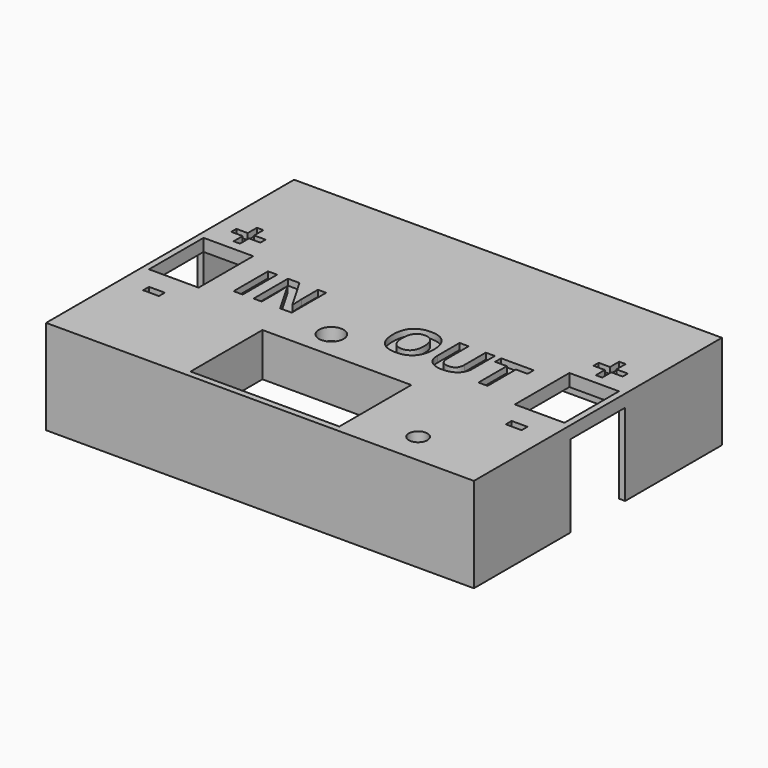
from build123d import *

# Parameters (mm, degrees)
F0_W         = 69
F0_H         = 50
F1_DEPTH     = 15.25
F0_R         = 2.5
F0_R_2       = 2
F0_R_3       = 1.5
F2_DEPTH     = 2
F3_DEPTH     = 13.25
F4_W         = 11
F4_H         = 13.25
F5_DEPTH     = 75
F6_DEPTH     = 7
F8_TEXT_SIZE = 9.7222222222
F9_DEPTH     = 1


# Not quite as in the source:
# - a feature names something its author has since deleted; it is built from what else it names
# - Text() gives the source's letters only with a copy of the font that has no kerning and outlines rounded to 1/6400 em; it was checked with that copy


with BuildPart() as f1:
    # F0 (on Top) → F1 (new body)
    with BuildSketch(Plane.XY):
        with Locations((2.621e-07, 0.3874345593)):
            Rectangle(F0_W, F0_H)
        Polygon((-33.4999997379, 5.8874345593), (-33.4999997379, 24.3874345593), (33.5000002621, 24.3874345593), (33.5000002621, 5.8874345593), (33.5000002621, -5.1125654407), (33.5000002621, -23.6125654407), (12.2500002621, -23.6125654407), (12.0000002621, -23.6125654407), (-11.9999997379, -23.6125654407), (-12.2499997379, -23.6125654407), (-33.4999997379, -23.6125654407), (-33.4999997379, -5.1125654407), align=None, mode=Mode.SUBTRACT)
    extrude(amount=-F1_DEPTH)

    # F0 (on Top) → F2 (join)
    with BuildSketch(Plane.XY):
        Polygon((33.5000002621, 24.3874345593), (-33.4999997379, 24.3874345593), (-33.4999997379, 5.8874345593), (-25.4999997379, 5.8874345593), (-25.4999997379, -5.1125654407), (-33.4999997379, -5.1125654407), (-33.4999997379, -23.6125654407), (-12.2499997379, -23.6125654407), (-12.2499997379, -8.6125654407), (12.2500002621, -8.6125654407), (12.2500002621, -23.6125654407), (33.5000002621, -23.6125654407), (33.5000002621, -5.1125654407), (25.5000002621, -5.1125654407), (25.5000002621, 5.8874345593), (33.5000002621, 5.8874345593), align=None)
        with Locations((-29.7499997379, -20.1125654407)):
            Circle(F0_R, mode=Mode.SUBTRACT)
        with Locations((-4.4999997379, -4.6125654407)):
            Circle(F0_R_2, mode=Mode.SUBTRACT)
        with Locations((21.5000002621, -19.6125654407)):
            Circle(F0_R_3, mode=Mode.SUBTRACT)
        with Locations((29.7500002621, -20.1125654407)):
            Circle(F0_R, mode=Mode.SUBTRACT)
        with Locations((-29.7499997379, 20.3874345593)):
            Circle(F0_R, mode=Mode.SUBTRACT)
        with Locations((29.7500002621, 20.3874345593)):
            Circle(F0_R, mode=Mode.SUBTRACT)
        with Locations((-29.7499997379, 20.3874345593)):
            Circle(F0_R)
        with Locations((-29.7499997379, 20.3874345593)):
            Circle(F0_R_3, mode=Mode.SUBTRACT)
        with Locations((29.7500002621, 20.3874345593)):
            Circle(F0_R)
        with Locations((29.7500002621, 20.3874345593)):
            Circle(F0_R_3, mode=Mode.SUBTRACT)
        with Locations((29.7500002621, -20.1125654407)):
            Circle(F0_R)
        with Locations((29.7500002621, -20.1125654407)):
            Circle(F0_R_3, mode=Mode.SUBTRACT)
        with Locations((-29.7499997379, -20.1125654407)):
            Circle(F0_R)
        with Locations((-29.7499997379, -20.1125654407)):
            Circle(F0_R_3, mode=Mode.SUBTRACT)
        with Locations((-29.7499997379, 20.3874345593)):
            Circle(F0_R_3)
        with Locations((29.7500002621, 20.3874345593)):
            Circle(F0_R_3)
        with Locations((29.7500002621, -20.1125654407)):
            Circle(F0_R_3)
        with Locations((-29.7499997379, -20.1125654407)):
            Circle(F0_R_3)
    extrude(amount=-F2_DEPTH)

    # F0 (on Top) → F3 (join)
    with BuildSketch(Plane.XY):
        with Locations((-29.7499997379, 20.3874345593)):
            Circle(F0_R)
        with Locations((-29.7499997379, 20.3874345593)):
            Circle(F0_R_3, mode=Mode.SUBTRACT)
        with Locations((29.7500002621, 20.3874345593)):
            Circle(F0_R)
        with Locations((29.7500002621, 20.3874345593)):
            Circle(F0_R_3, mode=Mode.SUBTRACT)
        with Locations((29.7500002621, -20.1125654407)):
            Circle(F0_R)
        with Locations((29.7500002621, -20.1125654407)):
            Circle(F0_R_3, mode=Mode.SUBTRACT)
        with Locations((-29.7499997379, -20.1125654407)):
            Circle(F0_R)
        with Locations((-29.7499997379, -20.1125654407)):
            Circle(F0_R_3, mode=Mode.SUBTRACT)
    extrude(amount=-F3_DEPTH)

    # F4 (on face) → F5 (cut)
    with BuildSketch(Plane.YZ.offset(34.5000002621)):
        with Locations((0.3874345593, -8.625)):
            Rectangle(F4_W, F4_H)
    extrude(amount=-F5_DEPTH, mode=Mode.SUBTRACT)


with BuildPart() as f6:
    # F0 (on Top) → F6 (new body)
    with BuildSketch(Plane.XY):
        Polygon((-12.2499997379, -8.6125654407), (-12.2499997379, -23.6125654407), (-11.9999997379, -23.6125654407), (-11.9999997379, -9.1125654407), (12.0000002621, -9.1125654407), (12.0000002621, -23.6125654407), (12.2500002621, -23.6125654407), (12.2500002621, -8.6125654407), align=None)
    extrude(amount=-F6_DEPTH)


with BuildPart() as f1_1:
    add(f1.part)

    # F7: union F6
    add(f6.part)

    # F8 (on face) → F9 (cut)
    with BuildSketch(Plane.XY):
        with Locations((-32.2206924293, 6.4316058829)):
            Text('+', F8_TEXT_SIZE, font='Open Sans', font_style=FontStyle.BOLD, text_align=(TextAlign.LEFT, TextAlign.BOTTOM))
        with Locations((-30.8034313603, -12.0420340896)):
            Text('-', F8_TEXT_SIZE, font='Open Sans', font_style=FontStyle.BOLD, text_align=(TextAlign.LEFT, TextAlign.BOTTOM))
        with Locations((-22.3314435763, -3.1136927819)):
            Text('IN', F8_TEXT_SIZE, font='Open Sans', font_style=FontStyle.BOLD, text_align=(TextAlign.LEFT, TextAlign.BOTTOM))
        with Locations((1.0156080334, -3.2976213766)):
            Text('OUT', F8_TEXT_SIZE, font='Open Sans', font_style=FontStyle.BOLD, text_align=(TextAlign.LEFT, TextAlign.BOTTOM))
        with Locations((26.2196836438, 6.4100607783)):
            Text('+', F8_TEXT_SIZE, font='Open Sans', font_style=FontStyle.BOLD, text_align=(TextAlign.LEFT, TextAlign.BOTTOM))
        with Locations((27.7056744562, -12.0713461824)):
            Text('-', F8_TEXT_SIZE, font='Open Sans', font_style=FontStyle.BOLD, text_align=(TextAlign.LEFT, TextAlign.BOTTOM))
    extrude(amount=-F9_DEPTH, mode=Mode.SUBTRACT)


solid = f1_1.part
